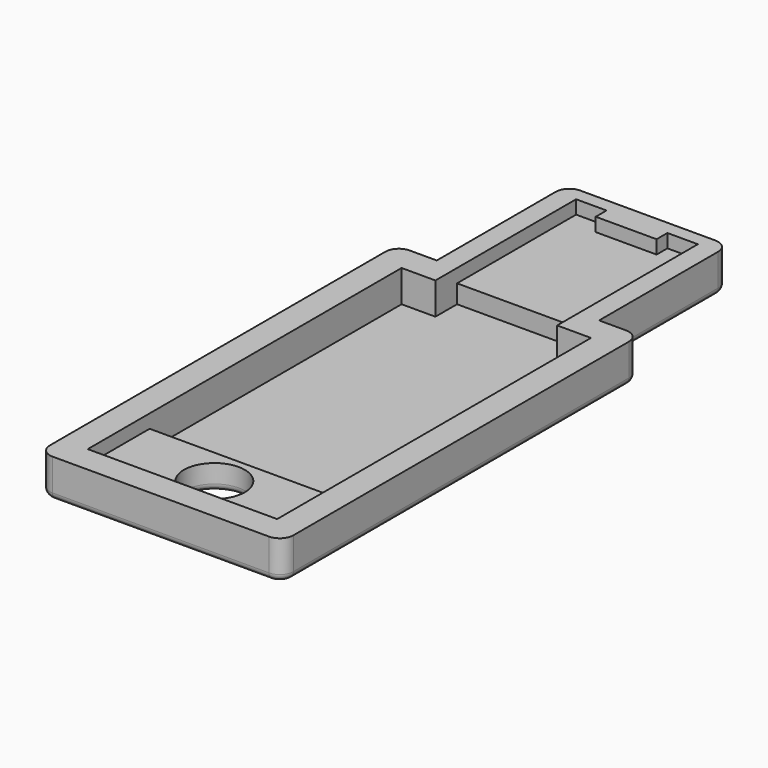
from build123d import *

# Parameters (mm, degrees)
F1_DEPTH = 2.36
F0_W     = 14
F0_H     = 5.7202167809
F0_R     = 2.25
F0_R_2   = 4.5
F2_DEPTH = 0.5
F3_R     = 0.49999
F4_DEPTH = 1.36
F5_DEPTH = 1.36


# Not quite as in the source:
# - a fillet or chamfer is up to 0.001 mm smaller than in the source, because OpenCascade refuses the exact size


with BuildPart() as f1:
    # F0 (on Top) → F1 (new body)
    with BuildSketch(Plane.XY):
        with BuildLine():
            ThreePointArc((-2, -1), (-1.7071067812, -1.7071067812), (-1, -2))
            Line((-1, -2), (15, -2))
            ThreePointArc((15, -2), (15.7071067812, -1.7071067812), (16, -1))
            Line((16, -1), (16, 30))
            ThreePointArc((16, 30), (15.7071067812, 30.7071067812), (15, 31))
            Line((15, 31), (13, 31))
            Line((13, 31), (13, 42))
            ThreePointArc((13, 42), (12.7071067812, 42.7071067812), (12, 43))
            Line((12, 43), (2, 43))
            ThreePointArc((2, 43), (1.2928932188, 42.7071067812), (1, 42))
            Line((1, 42), (1, 31))
            Line((1, 31), (-1, 31))
            ThreePointArc((-1, 31), (-1.7071067812, 30.7071067812), (-2, 30))
            Line((-2, 30), (-2, -1))
        make_face()
        Polygon((14, 0), (0, 0), (0, 5.7202167809), (0, 29), (2.5, 29), (2.5, 31), (2.5, 42), (4.75, 42), (4.75, 41), (9.25, 41), (9.25, 42), (11.5, 42), (11.5, 31), (11.5, 29), (14, 29), (14, 5.7202167809), align=None, mode=Mode.SUBTRACT)
    extrude(amount=F1_DEPTH)

    # F0 (on Top) → F2 (join)
    with BuildSketch(Plane.XY):
        with BuildLine():
            ThreePointArc((-2, -1), (-1.7071067812, -1.7071067812), (-1, -2))
            Line((-1, -2), (15, -2))
            ThreePointArc((15, -2), (15.7071067812, -1.7071067812), (16, -1))
            Line((16, -1), (16, 30))
            ThreePointArc((16, 30), (15.7071067812, 30.7071067812), (15, 31))
            Line((15, 31), (13, 31))
            Line((13, 31), (13, 42))
            ThreePointArc((13, 42), (12.7071067812, 42.7071067812), (12, 43))
            Line((12, 43), (2, 43))
            ThreePointArc((2, 43), (1.2928932188, 42.7071067812), (1, 42))
            Line((1, 42), (1, 31))
            Line((1, 31), (-1, 31))
            ThreePointArc((-1, 31), (-1.7071067812, 30.7071067812), (-2, 30))
            Line((-2, 30), (-2, -1))
        make_face()
        Polygon((14, 0), (0, 0), (0, 5.7202167809), (0, 29), (2.5, 29), (2.5, 31), (2.5, 42), (4.75, 42), (4.75, 41), (9.25, 41), (9.25, 42), (11.5, 42), (11.5, 31), (11.5, 29), (14, 29), (14, 5.7202167809), align=None, mode=Mode.SUBTRACT)
        with Locations((7, 2.8601083905)):
            Rectangle(F0_W, F0_H)
        with Locations((7, 2.95)):
            Circle(F0_R, mode=Mode.SUBTRACT)
        Polygon((2.5, 42), (2.5, 31), (11.5, 31), (11.5, 42), (9.25, 42), (9.25, 41), (4.75, 41), (4.75, 42), align=None)
        Polygon((0, 29), (0, 5.7202167809), (14, 5.7202167809), (14, 29), (11.5, 29), (11.5, 31), (2.5, 31), (2.5, 29), align=None)
        with Locations((7, 18.8)):
            Circle(F0_R_2, mode=Mode.SUBTRACT)
        with Locations((7, 18.8)):
            Circle(F0_R_2)
    extrude(amount=-F2_DEPTH)

    # F3 (radius 0.5 in the source; OpenCascade refuses exactly that, so slightly less here)
    f3_edges = [f1.edges().sort_by_distance(p)[0] for p in [
        (1, 36.5, -0.5),
        (0, 31, -0.5),
        (-1.707107, 30.707107, -0.5),
        (-2, 14.5, -0.5),
        (-1.707107, -1.707107, -0.5),
        (7, -2, -0.5),
        (15.707107, -1.707107, -0.5),
        (16, 14.5, -0.5),
        (15.707107, 30.707107, -0.5),
        (14, 31, -0.5),
        (13, 36.5, -0.5),
        (12.707107, 42.707107, -0.5),
        (7, 43, -0.5),
        (1.292893, 42.707107, -0.5),
        (4.75, 2.95, -0.5),
    ]]
    fillet(f3_edges, radius=F3_R)

    # F0 (on Top) → F4 (join)
    with BuildSketch(Plane.XY):
        Polygon((2.5, 42), (2.5, 31), (11.5, 31), (11.5, 42), (9.25, 42), (9.25, 41), (4.75, 41), (4.75, 42), align=None)
    extrude(amount=F4_DEPTH)

    # F0 (on Top) → F5 (join)
    with BuildSketch(Plane.XY):
        with Locations((7, 2.8601083905)):
            Rectangle(F0_W, F0_H)
        with Locations((7, 2.95)):
            Circle(F0_R, mode=Mode.SUBTRACT)
    extrude(amount=F5_DEPTH)


solid = f1.part
